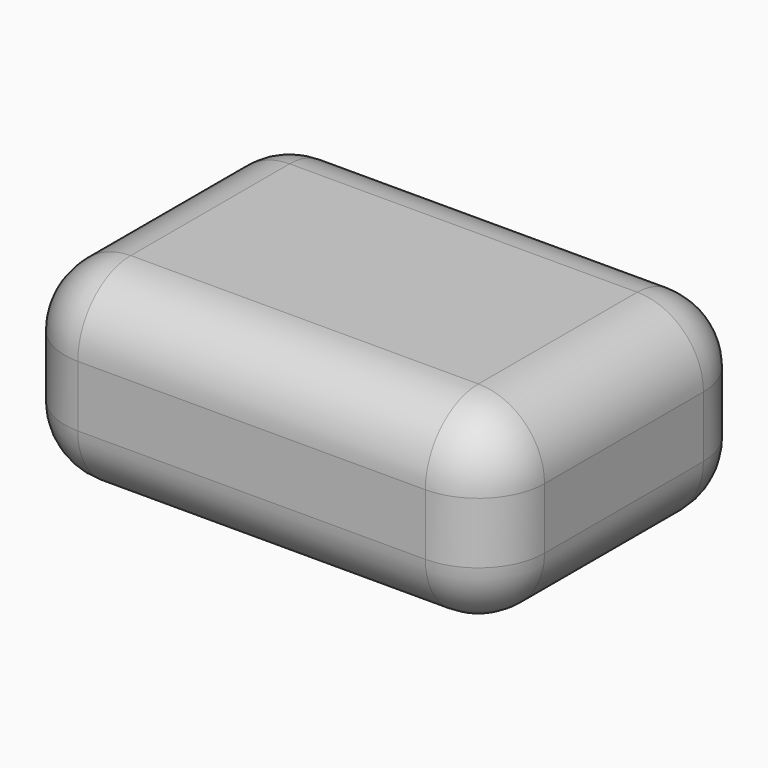
from build123d import *

# Parameters (mm, degrees)
F0_W     = 36.83
F0_H     = 25.4
F1_DEPTH = 14.859
F2_W     = 15.24
F2_H     = 4.699
F3_DEPTH = 18.542
F4_DEPTH = 16.256
F5_R     = 5.07999


# Not quite as in the source:
# - a fillet or chamfer is up to 0.001 mm smaller than in the source, because OpenCascade refuses the exact size


with BuildPart() as f1:
    # F0 (on Top) → F1 (new body)
    with BuildSketch(Plane.XY):
        Rectangle(F0_W, F0_H)
    extrude(amount=F1_DEPTH)

    # F2 (on Right) → F3 (cut)
    with BuildSketch(Plane.YZ):
        with Locations((0, 7.4295)):
            Rectangle(F2_W, F2_H)
    extrude(amount=-F3_DEPTH, mode=Mode.SUBTRACT)

    # F2 (on Right) → F4 (cut)
    with BuildSketch(Plane.YZ):
        with Locations((0, 7.4295)):
            Rectangle(F2_W, F2_H)
    extrude(amount=F4_DEPTH, mode=Mode.SUBTRACT)

    # F5 (radius 5.08 in the source; OpenCascade refuses exactly that, so slightly less here)
    f5_edges = [f1.edges().sort_by_distance(p)[0] for p in [
        (0, -12.7, 14.859),
        (18.415, 0, 14.859),
        (18.415, -12.7, 7.4295),
        (18.415, 0, 0),
        (18.415, 12.7, 7.4295),
        (0, 12.7, 0),
        (0, -12.7, 0),
        (0, 12.7, 14.859),
        (-18.415, 0, 14.859),
        (-18.415, 12.7, 7.4295),
        (-18.415, 0, 0),
        (-18.415, -12.7, 7.4295),
    ]]
    fillet(f5_edges, radius=F5_R)


solid = f1.part
